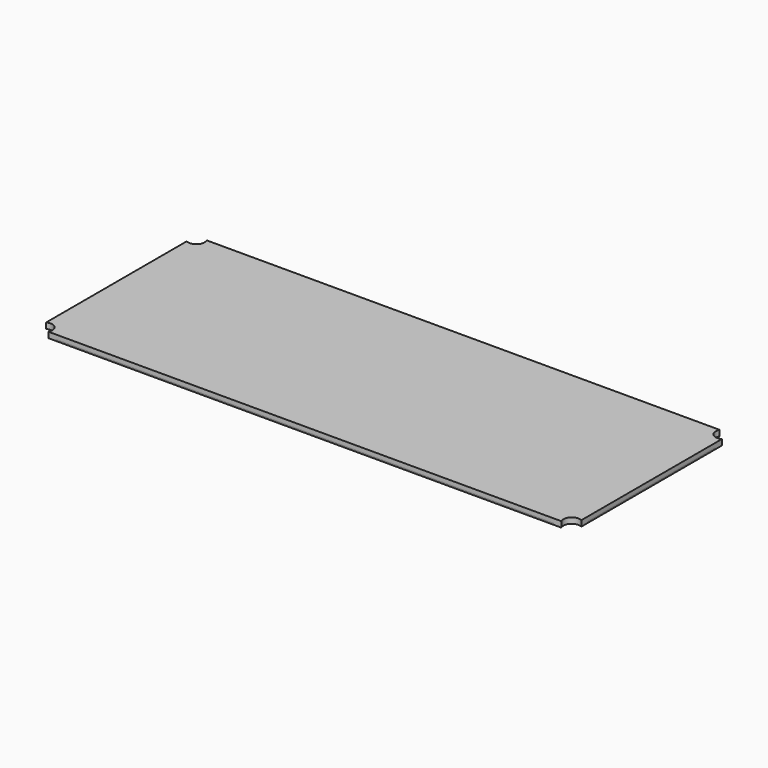
from build123d import *

# Parameters (mm, degrees)
F5_DEPTH = 12.7
F7_DEPTH = 3.175


# Not quite as in the source:
# - a length typed as a fraction of an inch, garbled in the dataset ("3 / 203.2 mm" for 3/8 in), is restored


with BuildPart() as f5:
    # F4 (on Top) → F5 (new body)
    with BuildSketch(Plane.XY):
        with BuildLine():
            Line((572.2333880236, 220.6625), (-572.2333880236, 220.6625))
            ThreePointArc((-572.2333880236, 220.6625), (-575.5229311857, 199.2854311857), (-596.9, 195.9958880236))
            Line((-596.9, 195.9958880236), (-596.9, -195.9958880236))
            ThreePointArc((-596.9, -195.9958880236), (-575.5229311857, -199.2854311857), (-572.2333880236, -220.6625))
            Line((-572.2333880236, -220.6625), (572.2333880236, -220.6625))
            ThreePointArc((572.2333880236, -220.6625), (575.5229311857, -199.2854311857), (596.9, -195.9958880236))
            Line((596.9, -195.9958880236), (596.9, 195.9958880236))
            ThreePointArc((596.9, 195.9958880236), (575.5229311857, 199.2854311857), (572.2333880236, 220.6625))
        make_face()
    extrude(amount=F5_DEPTH)


with BuildPart() as f7:
    # F6 (on Top) → F7 (new body)
    with BuildSketch(Plane.XY):
        Polygon((596.9, 177.9083623713), (554.1458623713, 220.6625), (-554.1458623713, 220.6625), (-596.9, 177.9083623713), (-596.9, -177.9083623713), (-554.1458623713, -220.6625), (554.1458623713, -220.6625), (596.9, -177.9083623713), align=None)
    extrude(amount=F7_DEPTH)


solid = Compound([f5.part, f7.part])
